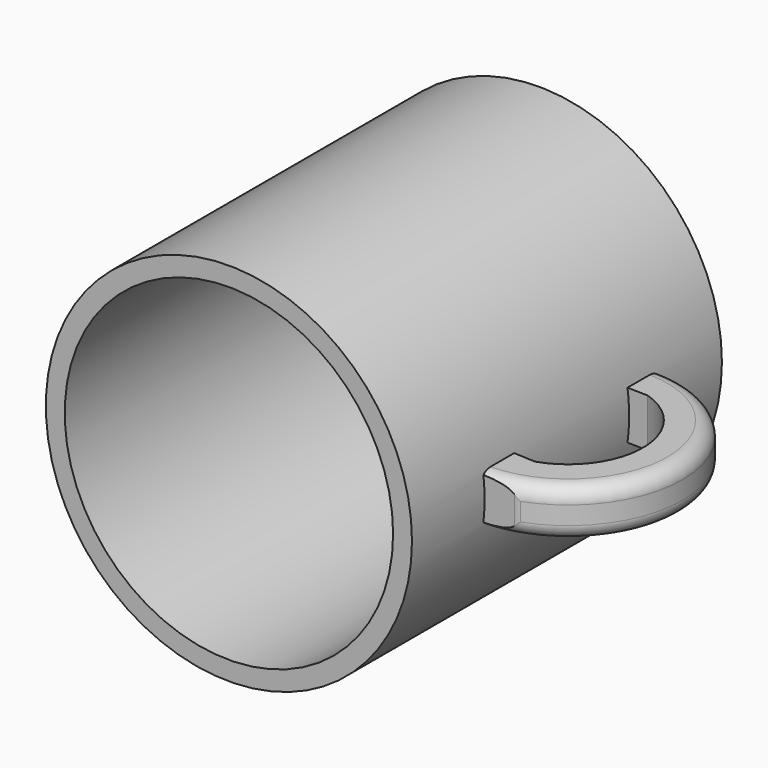
from build123d import *

# Parameters (mm, degrees)
F0_R         = 61.5738591245
F1_DEPTH     = 130.302
F2_T         = -6.35
F4_DEPTH     = 8.128
F5_T1_DEPTH  = 20.8040228352
F5_T3_DEPTH  = 20.562657233
F5_T8_ANGLE  = 182.1562701249
F5_S9_R      = 61.5738591245
F5_T10_DEPTH = 49
F5_T14_ANGLE = 182.1562701249
F5_S15_R     = 61.5738591245
F5_T16_DEPTH = 49


# Not quite as in the source:
# - a fillet or chamfer that OpenCascade refuses, or shapes differently, is made with other operations: its cross-section is extruded or revolved along the edge and cut away or added


with BuildPart() as f1:
    # F0 (on Front) → F1 (new body)
    with BuildSketch(Plane.XZ):
        Circle(F0_R)
    extrude(amount=F1_DEPTH)

    # F2
    f2_openings = [f1.faces().sort_by_distance(p)[0] for p in [
        (0, -130.302, 0),
    ]]
    offset(amount=F2_T, openings=f2_openings)

    # F3 (on Top) → F4 (join, symmetric)
    with BuildSketch(Plane.XY):
        with BuildLine():
            Line((59.0887926519, -99.7823445332), (72.4941612439, -99.7823445332))
            ThreePointArc((72.4941612439, -99.7823445332), (98.9458486723, -62.8559772667), (71.8830453985, -26.3751186382))
            Line((71.8830453985, -26.3751186382), (59.0614564717, -26.3751186382))
            Line((59.0614564717, -26.3751186382), (59.0614564717, -38.9808338419))
            Line((59.0614564717, -38.9808338419), (67.8895905633, -39.1665116223))
            ThreePointArc((67.8895905633, -39.1665116223), (85.5460362932, -62.9675308307), (68.2882977353, -87.0592109513))
            Line((68.2882977353, -87.0592109513), (59.0887926519, -86.546982936))
            Line((59.0887926519, -86.546982936), (59.0887926519, -99.7823445332))
        make_face()
    extrude(amount=F4_DEPTH, both=True)

    # F5: fillet of radius 5.08 on 4 edges, made by hand

    # F5_s2 → F5_t1 (cut)
    with BuildSketch(Plane.XY.offset(-10.4020114176)):
        with BuildLine():
            ThreePointArc((71.6465994249, -99.7823445332), (72.5131887158, -99.7078837649), (73.3543737137, -99.4866842973))
            ThreePointArc((73.3543737137, -99.4866842973), (72.925139457, -99.6370514033), (72.4941612439, -99.7823445332))
            Line((72.4941612439, -99.7823445332), (71.6465994249, -99.7823445332))
        make_face()
    extrude(amount=F5_T1_DEPTH, mode=Mode.SUBTRACT)

    # F5_s4 → F5_t3 (cut)
    with BuildSketch(Plane.XY.offset(-10.2813286165)):
        with BuildLine():
            ThreePointArc((71.0804640636, -26.3751186382), (71.9022151056, -26.4420232646), (72.7023208932, -26.6409748489))
            ThreePointArc((72.7023208932, -26.6409748489), (72.2934256102, -26.5057587291), (71.8830453985, -26.3751186382))
            Line((71.8830453985, -26.3751186382), (71.0804640636, -26.3751186382))
        make_face()
    extrude(amount=F5_T3_DEPTH, mode=Mode.SUBTRACT)


with BuildPart() as f5_tool6:
    # F5_s7 → F5_t8 (revolve)
    with BuildSketch(Plane(origin=(61.0497406785, -0.6405689566, 0), x_dir=(0, 0, 1), z_dir=(-0.9999449575, 0.010491997, 0))):
        with BuildLine():
            ThreePointArc((-8.128, -96.0134100137), (-6.6401024484, -99.6055124621), (-3.048, -101.0934100137))
            Line((-3.048, -101.0934100137), (-8.128, -101.0934100137))
            Line((-8.128, -101.0934100137), (-8.128, -96.0134100137))
        make_face()
    revolve(axis=Axis((60.393573296, -63.1769253215, -8.128), (0, 0, 1)), revolution_arc=F5_T8_ANGLE)

    # F5_s9 → F5_t10 (cut, symmetric)
    with BuildSketch(Plane.XZ.offset(63.2)):
        Circle(F5_S9_R)
    extrude(amount=F5_T10_DEPTH, both=True, mode=Mode.SUBTRACT)


with BuildPart() as f1_1:
    add(f1.part)

    # F5_t5: cut F5_tool6
    add(f5_tool6.part, mode=Mode.SUBTRACT)


with BuildPart() as f5_tool12:
    # F5_s13 → F5_t14 (revolve)
    with BuildSketch(Plane(origin=(61.0497406785, -0.6405689566, 0), x_dir=(0, 0, 1), z_dir=(-0.9999449575, 0.010491997, 0))):
        with BuildLine():
            ThreePointArc((8.128, -96.0134100137), (6.6401024484, -99.6055124621), (3.048, -101.0934100137))
            Line((3.048, -101.0934100137), (8.128, -101.0934100137))
            Line((8.128, -101.0934100137), (8.128, -96.0134100137))
        make_face()
    revolve(axis=Axis((60.393573296, -63.1769253215, 8.128), (0, 0, 1)), revolution_arc=F5_T14_ANGLE)

    # F5_s15 → F5_t16 (cut, symmetric)
    with BuildSketch(Plane.XZ.offset(63.2)):
        Circle(F5_S15_R)
    extrude(amount=F5_T16_DEPTH, both=True, mode=Mode.SUBTRACT)


with BuildPart() as f1_2:
    add(f1_1.part)

    # F5_t11: cut F5_tool12
    add(f5_tool12.part, mode=Mode.SUBTRACT)


solid = f1_2.part
